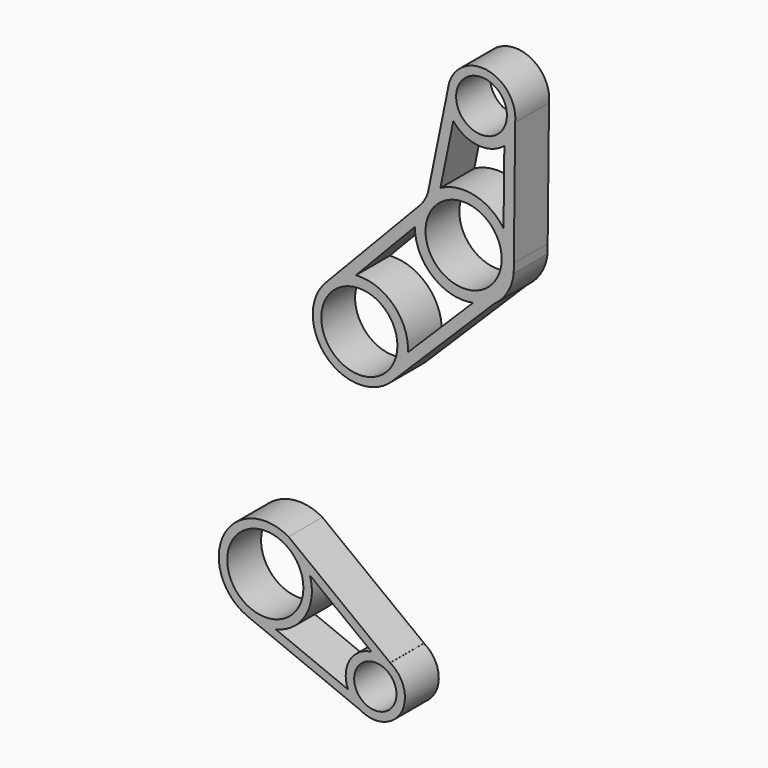
from build123d import *

# Parameters (mm, degrees)
F0_R        = 5
F0_R_2      = 9
F1_DEPTH    = 10
F2_T        = -2
F0_R_3      = 6
F3_DEPTH    = 10
F4_T        = 2.5
F4_T3_DEPTH = 15


# Not quite as in the source:
# - a shell that OpenCascade refuses in one call is made with other operations: the cavity is built on its own and cut out


with BuildPart() as f1:
    # F0 (on Front) → F1 (new body)
    with BuildSketch(Plane.XZ):
        with BuildLine():
            Line((-8.8314399067, -49.4378021172), (-32.8488921378, -31.037019376))
            ThreePointArc((-32.8488921378, -31.037019376), (-48.2033224661, -35.6963509232), (-42.5721099109, -50.7215745931))
            Line((-42.5721099109, -50.7215745931), (-15.8328549722, -61.6009637621))
            ThreePointArc((-15.8328549722, -61.6009637621), (-6.2740037455, -59.026402979), (-8.8485645285, -49.4675517523))
            Line((-8.8485645285, -49.4675517523), (-8.8314399067, -49.4378021172))
        make_face()
        with Locations((-12.3407097504, -55.5342577572)):
            Circle(F0_R, mode=Mode.SUBTRACT)
        with Locations((-38.3408783427, -40.5679210922)):
            Circle(F0_R_2, mode=Mode.SUBTRACT)
    extrude(amount=F1_DEPTH)

    # F2: a shell. OpenCascade refuses it in one call, so the cavity is built on its own and cut out:
    # the body offset inwards by the wall thickness, plus a prism from it out through each open face.
    f2_core = offset(f1.part, amount=F2_T, mode=Mode.PRIVATE)
    f2_exits = [f2_core.faces().sort_by_distance(p)[0] for p in [
        (-23.974872, -8, -48.858148),
        (-23.974872, -2, -48.858148),
    ]]
    add(f2_core, mode=Mode.SUBTRACT)
    extrude(f2_exits, amount=-F2_T, mode=Mode.SUBTRACT)


with BuildPart() as f3:
    # F0 (on Front) → F3 (new body)
    with BuildSketch(Plane.XZ):
        with BuildLine():
            Line((-1.8184846325, 48.0031181659), (-24.0760708981, 24.6802065861))
            ThreePointArc((-24.0760708981, 24.6802065861), (-23.8168254633, 9.2289086893), (-8.3634526675, 9.2844435787))
            Line((-8.3634526675, 9.2844435787), (15.7316601136, 33.2355234732))
            ThreePointArc((15.7316601136, 33.2355234732), (18.901820518, 36.6574412714), (20.3688188047, 41.0854605164))
            Line((20.3688188047, 41.0854605164), (20.3915449047, 43.1814512794))
            Line((20.3915449047, 43.1814512794), (20.7101995844, 72.5704474305))
            ThreePointArc((20.7101995844, 72.5704474305), (13.6038459907, 81.3738410149), (4.8004524063, 74.2674874211))
            Line((4.8004524063, 74.2674874211), (0.2318668126, 51.9236662992))
            ThreePointArc((0.2318668126, 51.9236662992), (-0.5168921946, 49.8188330045), (-1.8184846325, 48.0031181659))
        make_face()
        with Locations((-16.1182750016, 17.0859005302)):
            Circle(F0_R_2, mode=Mode.SUBTRACT)
        with Locations((8.5178585723, 43.0951789021)):
            Circle(F0_R_2, mode=Mode.SUBTRACT)
        with Locations((12.7553259954, 73.4189674258)):
            Circle(F0_R_3, mode=Mode.SUBTRACT)
    extrude(amount=F3_DEPTH)

    # F4: shell of thickness 2.5, made by hand


with BuildPart() as f4_core1:
    # F4_t2: copy of F3
    add(f3.part)

    # the walls: a layer under each face that stays
    f4_faces = [f4_core1.faces().sort_by_distance(p)[0] for p in [
        (18.901820518, -5, 36.6574412714),
        (6.7553259954, -5, 73.4189674258),
        (-0.4821414277, -5, 43.0951789021),
        (-25.1182750016, -5, 17.0859005302),
        (-23.8168254633, -5, 9.2289086893),
        (-12.9472777653, -5, 36.341662376),
        (-0.5168921946, -5, 49.8188330045),
        (2.5161596095, -5, 63.0955768602),
        (13.6038459907, -5, 81.3738410149),
        (20.5395091946, -5, 56.8279539735),
        (3.684103723, -5, 21.259983526),
    ]]
    thicken(f4_faces, amount=-F4_T, mode=Mode.SUBTRACT)

    # F4_s4 → F4_t3 (cut)
    with BuildSketch(Plane.XZ.offset(-2.5)):
        Polygon((15.7636046927, 33.1973004983), (14.2996618195, 35.2847625725), (14.1224923885, 35.1609574377), (13.9692004922, 35.0085818713), align=None)
        Polygon((4.7511001784, 74.2751471197), (7.2497772094, 73.7666800637), (7.27368954, 73.8836293527), (7.2863504029, 74.0023249226), align=None)
        Polygon((20.760057095, 72.5675247552), (18.2243015879, 72.8356099291), (18.2116407249, 72.7169143592), (18.2103465254, 72.5975524692), align=None)
    extrude(amount=F4_T3_DEPTH, mode=Mode.SUBTRACT)


with BuildPart() as f3_1:
    add(f3.part)

    # what is left inside the walls is the cavity
    f4_cavity = [f4_core1.part.solids().sort_by_distance(p)[0] for p in [
        (-3.08156, -0.025, 25.399802),
        (18.029816, -6.666667, 58.253404),
    ]]
    add(f4_cavity, mode=Mode.SUBTRACT)


solid = Compound([f1.part, f3_1.part])
